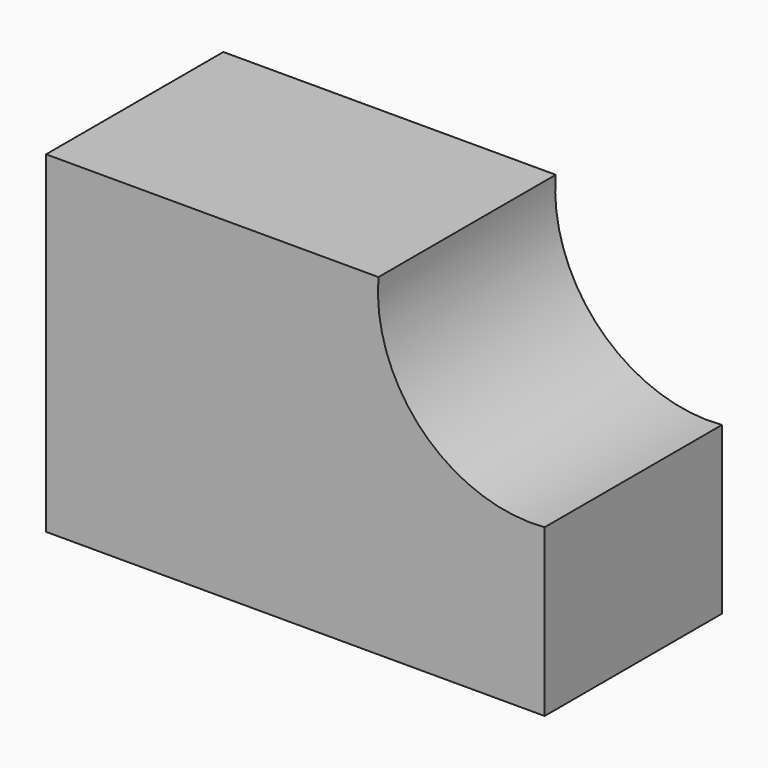
from build123d import *

# Parameters (mm, degrees)
F0_W     = 57.15
F0_H     = 38.1
F1_DEPTH = 25.4
F3_DEPTH = 25.4
F4_W     = 15.0772607885
F4_H     = 19.0978627652
F5_DEPTH = 107
F7_DEPTH = 107
F8_W     = 12.6649001613
F8_H     = 19.2988961935
F9_DEPTH = 107


# Not quite as in the source:
# - an extrude ends at something that could not be found from the text; its depth is read off the source's solid


with BuildPart() as f1:
    # F0 (on Front) → F1 (new body)
    with BuildSketch(Plane.XZ):
        with Locations((28.575, 19.05)):
            Rectangle(F0_W, F0_H)
    extrude(amount=F1_DEPTH)

    # F2 (on face) → F3 (cut)
    with BuildSketch(Plane.XZ.offset(25.4)):
        with BuildLine():
            Line((57.15, 38.1), (38.1, 38.1))
            ThreePointArc((38.1, 38.1), (43.2045261365, 24.1545261365), (57.15, 19.05))
            Line((57.15, 19.05), (57.15, 38.1))
        make_face()
    extrude(amount=-F3_DEPTH, mode=Mode.SUBTRACT)

    # F4 (on Right) → F5 (cut, through all)
    with BuildSketch(Plane.YZ):
        with Locations((-12.0618094224, 28.9483414963)):
            Rectangle(F4_W, F4_H)
    extrude(amount=-F5_DEPTH, mode=Mode.SUBTRACT)

    # F6 (on Right) → F7 (cut, through all)
    with BuildSketch(Plane.YZ):
        Polygon((-6.7345094867, 37.8941856325), (-18.3942597359, 38.2962450385), (-18.3942597359, 24.6261935681), (-6.7345094867, 24.6261935681), align=None)
    extrude(amount=-F7_DEPTH, mode=Mode.SUBTRACT)

    # F8 (on Right) → F9 (cut, through all)
    with BuildSketch(Plane.YZ):
        with Locations((-11.2576889805, 28.6467969418)):
            Rectangle(F8_W, F8_H)
    extrude(amount=-F9_DEPTH, mode=Mode.SUBTRACT)


solid = f1.part
